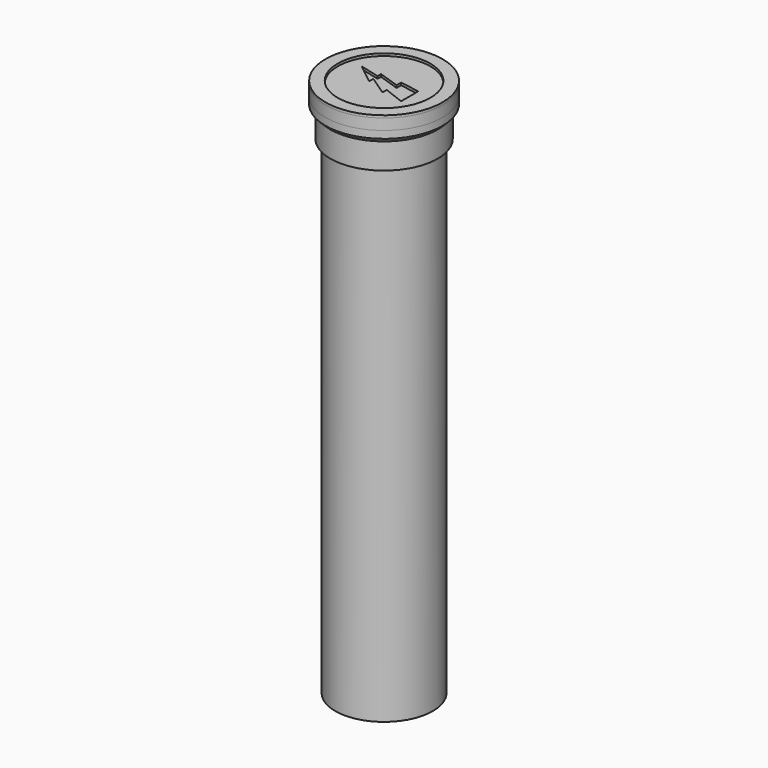
from build123d import *

# Parameters (mm, degrees)
F2_R         = 20
F3_DEPTH     = 200
F6_DEPTH     = 1
F5_R         = 24
F5_R_2       = 19
F7_DEPTH     = 1
F8_R         = 20.25
F9_DEPTH     = 16
F10_S5_R     = 24
F10_T6_DEPTH = 40


# Not quite as in the source:
# - a fillet or chamfer that OpenCascade refuses, or shapes differently, is made with other operations: its cross-section is extruded or revolved along the edge and cut away or added


with BuildPart() as f1:
    # F0 (on Front) → F1 (revolve)
    with BuildSketch(Plane.XZ):
        Polygon((-22, 0), (-20, 0), (0, 0), (0, 20), (-22, 20), (-24, 20), (-24, 15.5146932229), (-22, 15.5146932229), align=None)
    revolve(axis=Axis((0, 0, 10), (0, 0, -1)))

    # F5 (on face) → F6 (cut)
    with BuildSketch(Plane.XY.offset(20)):
        Polygon((11.9780020788, -6.2227640148), (11.9780020788, 2.6007659641), (3.8897663796, 3.8612704928), (3.8897663796, 1.5650035572), (-4.8287207231, 4.4915222406), (-4.8287207231, 2.705808496), (-13.0219979212, 4.8066484589), (-4.6587968989, -1.829864401), (-4.6587968989, 0.3787560728), (3.4695986625, -5.1723431725), (3.4695986625, -2.9664605056), align=None)
    extrude(amount=-F6_DEPTH, mode=Mode.SUBTRACT)

    # F5 (on face) → F7 (join)
    with BuildSketch(Plane.XY.offset(20)):
        Circle(F5_R)
        Circle(F5_R_2, mode=Mode.SUBTRACT)
    extrude(amount=F7_DEPTH)

    # F8 (on face) → F9 (cut)
    with BuildSketch(Plane(origin=(0, 0, 0), x_dir=(1, 0, 0), z_dir=(0, 0, -1))):
        Circle(F8_R)
    extrude(amount=-F9_DEPTH, mode=Mode.SUBTRACT)

    # F10: chamfer of 5 on 1 edges, made by hand


with BuildPart() as f3:
    # F2 (on Top) → F3 (new body)
    with BuildSketch(Plane.XY):
        Circle(F2_R)
    extrude(amount=-F3_DEPTH)


with BuildPart() as f10_tool2:
    # F10_s3 → F10_t4 (revolve)
    with BuildSketch(Plane.XZ):
        Polygon((-22, 10.5146932229), (-27, 15.5146932229), (-22, 15.5146932229), align=None)
    revolve(axis=Axis((0, 0, 15.5146932229), (0, 0, -1)))

    # F10_s5 → F10_t6 (intersect, symmetric)
    with BuildSketch(Plane.XY.offset(13)):
        Circle(F10_S5_R)
    extrude(amount=F10_T6_DEPTH, both=True, mode=Mode.INTERSECT)


with BuildPart() as f1_1:
    add(f1.part)

    # F10_t1: union F10_tool2
    add(f10_tool2.part)


solid = Compound([f3.part, f1_1.part])
